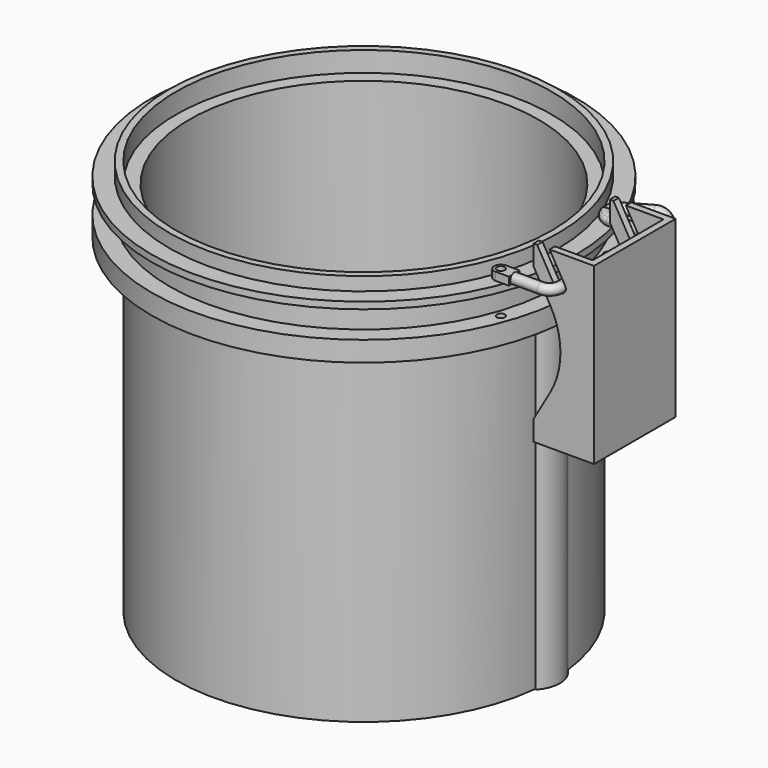
from build123d import *

# Parameters (mm, degrees)
F2_R           = 3.81
F3_DEPTH       = 57.151
F4_R           = 3.81
F5_DEPTH       = 7.62
F11_R          = 4.7625
F15_R          = 3.81
F16_DEPTH      = 122.8735001
F16_DEPTH_BACK = 12.701
F20_DEPTH      = 304.8
F22_DEPTH      = 88.9
F22_DEPTH_BACK = 76.2
F24_DEPTH      = 96.52


with BuildPart() as f1:
    # F0 (on Front) → F1 (revolve)
    with BuildSketch(Plane.XZ):
        Polygon((0, 25.4), (0, 0), (6.35, 0), (6.35, 19.05), (19.05, 19.05), (19.05, 6.35), (22.86, 6.35), (22.86, 25.4), (6.35, 25.4), (6.35, 50.8), (22.86, 50.8), (22.86, 57.15), (6.35, 57.15), (6.35, 69.85), (0, 69.85), (0, 50.8), align=None)
    revolve(axis=Axis((-177.8, 0, 29.9224383198), (0, 0, 1)))

    # F2 (on face) → F3 (cut, through all)
    with BuildSketch(Plane.XY.offset(57.15)):
        with Locations((2.54, -63.5)):
            Circle(F2_R)
        with Locations((2.54, 63.5)):
            Circle(F2_R)
    extrude(amount=-F3_DEPTH, mode=Mode.SUBTRACT)

    # F17 (on Front) → F18 (revolve)
    with BuildSketch(Plane.XZ):
        Polygon((0, -304.8), (0, 0), (0, 50.8), (-12.7, 50.8), (-12.7, -304.8), align=None)
    revolve(axis=Axis((-177.8, 0, 69.85), (0, 0, -1)))


with BuildPart() as f5:
    # F4 (on face) → F5 (new body)
    with BuildSketch(Plane.XY.offset(57.15)):
        with BuildLine():
            Line((15.24, -69.85), (15.24, -57.15))
            Line((15.24, -57.15), (2.54, -57.15))
            ThreePointArc((2.54, -57.15), (-3.81, -63.5), (2.54, -69.85))
            Line((2.54, -69.85), (15.24, -69.85))
        make_face()
        with Locations((2.54, -63.5)):
            Circle(F4_R, mode=Mode.SUBTRACT)
    extrude(amount=F5_DEPTH)

    # F10: sweep along a path in F9
    with BuildLine(Plane.XY.offset(60.96)) as f10_path:
        Line((15.24, -63.5), (40.64, -63.5))
        ThreePointArc((40.64, -63.5), (47.8242048969, -60.5242048969), (50.8, -53.34))
        Line((50.8, -53.34), (50.8, 43.18))
        ThreePointArc((50.8, 43.18), (47.8242048969, 50.3642048969), (40.64, 53.34))
        Line((40.64, 53.34), (12.7, 53.34))
        ThreePointArc((12.7, 53.34), (5.5157951031, 56.3157951031), (2.54, 63.5))
        ThreePointArc((2.54, 63.5), (3.9011818976, 68.58), (7.62, 72.2988181024))
        Line((7.62, 72.2988181024), (29.6170452561, 84.9988181024))
    # F6 (on face) → F10 (sweep)
    with BuildSketch(Plane.YZ.offset(15.24)):
        with BuildLine():
            Line((-66.3575, 64.77), (-60.6425, 64.77))
            ThreePointArc((-60.6425, 64.77), (-63.5, 65.7225), (-66.3575, 64.77))
        make_face()
        with BuildLine():
            ThreePointArc((-60.6425, 57.15), (-59.2402905029, 58.8301452514), (-58.7375, 60.96))
            ThreePointArc((-58.7375, 60.96), (-59.2402905029, 63.0898547486), (-60.6425, 64.77))
            Line((-60.6425, 64.77), (-66.3575, 64.77))
            ThreePointArc((-66.3575, 64.77), (-68.2625, 60.96), (-66.3575, 57.15))
            Line((-66.3575, 57.15), (-60.6425, 57.15))
        make_face()
        with BuildLine():
            ThreePointArc((-66.3575, 57.15), (-63.5, 56.1975), (-60.6425, 57.15))
            Line((-60.6425, 57.15), (-66.3575, 57.15))
        make_face()
    sweep(path=f10_path.line)

    # F14: sweep along a path in F13
    with BuildLine(Plane(origin=(-29.4013065702, 50.9245567884, 0), x_dir=(0.8660254038, 0.5, 0), z_dir=(0.5, -0.8660254038, 0))) as f14_path:
        ThreePointArc((68.1485226281, 60.96), (75.3327275249, 57.9842048969), (78.3085226281, 50.8))
        Line((78.3085226281, 50.8), (78.3085226281, -50.8))
        ThreePointArc((78.3085226281, -50.8), (75.3327275249, -57.9842048969), (68.1485226281, -60.96))
        Line((68.1485226281, -60.96), (55.4485226281, -60.96))
    # F11 (on face) → F14 (sweep)
    with BuildSketch(Plane(origin=(59.0183518263, 34.074261314, 0), x_dir=(-0.5, 0.8660254038, 0), z_dir=(0.8660254038, 0.5, 0))):
        with Locations((58.8026131403, 60.96)):
            Circle(F11_R)
    sweep(path=f14_path.line)

    # F15 (on face) → F16 (cut, two sides)
    with BuildSketch(Plane.XY.offset(57.15)) as f16_sk:
        with Locations((2.54, 63.5)):
            Circle(F15_R)
    extrude(amount=-F16_DEPTH, mode=Mode.SUBTRACT)
    extrude(f16_sk.sketch, amount=F16_DEPTH_BACK, mode=Mode.SUBTRACT)


with BuildPart() as f20:
    # F19 (on face) → F20 (new body, through all)
    with BuildSketch(Plane(origin=(0, 0, 0), x_dir=(1, 0, 0), z_dir=(0, 0, -1))):
        with BuildLine():
            Line((0, 19.05), (0, 0))
            Line((0, 0), (0, -19.05))
            ThreePointArc((0, -19.05), (7.62, 0), (0, 19.05))
        make_face()
    extrude(amount=F20_DEPTH)


with BuildPart() as f22:
    # F21 (on Top) → F22 (new body, two sides)
    with BuildSketch(Plane.XY) as f22_sk:
        Polygon((82.5499994576, -53.34), (82.5499994576, -5.08), (82.5499994576, 43.18), (25.3999994576, 43.18), (25.3999994576, 36.8300005424), (76.2, 36.8300005424), (76.2, -5.08), (76.2, -46.9900005424), (25.3999994576, -46.9900005424), (25.3999994576, -53.34), align=None)
    extrude(amount=F22_DEPTH)
    extrude(f22_sk.sketch, amount=-F22_DEPTH_BACK)

    # F23 (on face) → F24 (cut, through all)
    with BuildSketch(Plane.XZ.offset(53.34)):
        with BuildLine():
            ThreePointArc((46.4005909488, 58.42), (52.1148007491, 56.0530968025), (55.88, 60.96))
            ThreePointArc((55.88, 60.96), (55.7069031975, 62.2748007491), (55.1994090512, 63.5))
            ThreePointArc((55.1994090512, 63.5), (48.26, 65.3594090512), (46.4005909488, 58.42))
        make_face()
        with BuildLine():
            ThreePointArc((46.4005909488, 58.42), (48.26, 65.3594090512), (55.1994090512, 63.5))
            Line((55.1994090512, 63.5), (40.5347122138, 88.9))
            Line((40.5347122138, 88.9), (28.8029547439, 88.9))
            Line((28.8029547439, 88.9), (46.4005909488, 58.42))
        make_face()
        with BuildLine():
            Line((41.0470447137, 42.7485226281), (25.3999994576, 69.85))
            Line((25.3999994576, 69.85), (25.3999994576, -57.15))
            Line((25.3999994576, -57.15), (41.0470447137, -30.0485226281))
            ThreePointArc((41.0470447137, -30.0485226281), (48.3195002919, -12.4912617395), (50.7999994576, 6.35))
            ThreePointArc((50.7999994576, 6.35), (48.3195002919, 25.1912617395), (41.0470447137, 42.7485226281))
        make_face()
    extrude(amount=-F24_DEPTH, mode=Mode.SUBTRACT)


solid = Compound([f1.part, f5.part, f20.part, f22.part])
